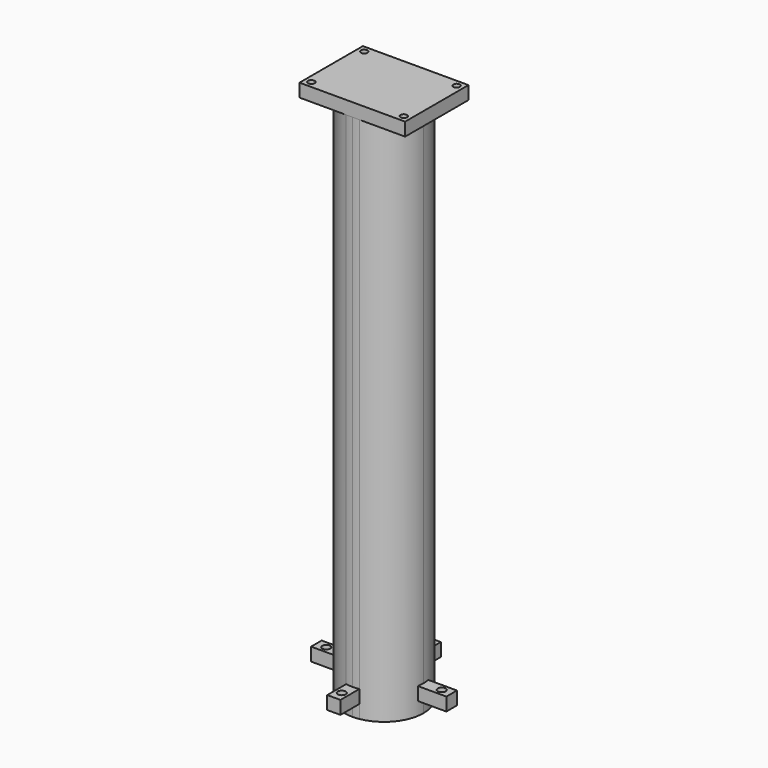
from build123d import *

# Parameters (mm, degrees)
F0_R     = 5
F1_DEPTH = 20
F2_DEPTH = 800
F5_DEPTH = 10
F6_DEPTH = 10
F0_R_2   = 6
F7_DEPTH = 956


# Not quite as in the source:
# - a feature names something its author has since deleted; it is built from what else it names


with BuildPart() as f1:
    # F0 (on Top) → F1 (new body)
    with BuildSketch(Plane.XY):
        with BuildLine():
            ThreePointArc((-59.160797831, 10), (-42.4264068712, 42.4264068712), (-10, 59.160797831))
            Line((-10, 59.160797831), (-10, 60))
            Line((-10, 60), (-80, 60))
            Line((-80, 60), (-80, 10))
            Line((-80, 10), (-59.160797831, 10))
        make_face()
        with Locations((-70, 50)):
            Circle(F0_R, mode=Mode.SUBTRACT)
        with BuildLine():
            ThreePointArc((59.160797831, -10), (59.7898313673, -5.0175756168), (60, 0))
            ThreePointArc((60, 0), (59.7898313673, 5.0175756168), (59.160797831, 10))
            ThreePointArc((59.160797831, 10), (42.4264068712, 42.4264068712), (10, 59.160797831))
            ThreePointArc((10, 59.160797831), (5.0175756193, 59.7898313671), (5e-09, 60))
            ThreePointArc((5e-09, 60), (-5.0175756143, 59.7898313675), (-10, 59.160797831))
            ThreePointArc((-10, 59.160797831), (-42.4264068712, 42.4264068712), (-59.160797831, 10))
            ThreePointArc((-59.160797831, 10), (-60, 0), (-59.160797831, -10))
            ThreePointArc((-59.160797831, -10), (-42.4264068712, -42.4264068712), (-10, -59.160797831))
            ThreePointArc((-10, -59.160797831), (-5.0175756489, -59.7898313646), (-6.44e-08, -60))
            ThreePointArc((-6.44e-08, -60), (5.0175755847, -59.78983137), (10, -59.160797831))
            ThreePointArc((10, -59.160797831), (42.4264068712, -42.4264068712), (59.160797831, -10))
        make_face()
        with BuildLine():
            ThreePointArc((10, 59.160797831), (42.4264068712, 42.4264068712), (59.160797831, 10))
            Line((59.160797831, 10), (80, 10))
            Line((80, 10), (80, 60))
            Line((80, 60), (10, 60))
            Line((10, 60), (10, 59.160797831))
        make_face()
        with Locations((70, 50)):
            Circle(F0_R, mode=Mode.SUBTRACT)
        with BuildLine():
            ThreePointArc((59.160797831, 10), (59.7898313673, 5.0175756168), (60, 0))
            ThreePointArc((60, 0), (59.7898313673, -5.0175756168), (59.160797831, -10))
            Line((59.160797831, -10), (80, -10))
            Line((80, -10), (80, 10))
            Line((80, 10), (59.160797831, 10))
        make_face()
        with BuildLine():
            Line((80, -10), (59.160797831, -10))
            ThreePointArc((59.160797831, -10), (42.4264068712, -42.4264068712), (10, -59.160797831))
            Line((10, -59.160797831), (10, -60))
            Line((10, -60), (80, -60))
            Line((80, -60), (80, -10))
        make_face()
        with Locations((70, -50)):
            Circle(F0_R, mode=Mode.SUBTRACT)
        with BuildLine():
            ThreePointArc((-59.160797831, -10), (-60, 0), (-59.160797831, 10))
            Line((-59.160797831, 10), (-80, 10))
            Line((-80, 10), (-80, -10))
            Line((-80, -10), (-59.160797831, -10))
        make_face()
        with BuildLine():
            Line((-10, -60), (-10, -59.160797831))
            ThreePointArc((-10, -59.160797831), (-42.4264068712, -42.4264068712), (-59.160797831, -10))
            Line((-59.160797831, -10), (-80, -10))
            Line((-80, -10), (-80, -60))
            Line((-80, -60), (-10, -60))
        make_face()
        with Locations((-70, -50)):
            Circle(F0_R, mode=Mode.SUBTRACT)
        with BuildLine():
            Line((-10, -60), (-6.44e-08, -60))
            ThreePointArc((-6.44e-08, -60), (-5.0175756489, -59.7898313646), (-10, -59.160797831))
            Line((-10, -59.160797831), (-10, -60))
        make_face()
        with BuildLine():
            Line((10, -60), (10, -59.160797831))
            ThreePointArc((10, -59.160797831), (5.0175755847, -59.78983137), (-6.44e-08, -60))
            Line((-6.44e-08, -60), (10, -60))
        make_face()
        with BuildLine():
            ThreePointArc((-10, 59.160797831), (-5.0175756143, 59.7898313675), (5e-09, 60))
            Line((5e-09, 60), (-10, 60))
            Line((-10, 60), (-10, 59.160797831))
        make_face()
        with BuildLine():
            ThreePointArc((5e-09, 60), (5.0175756193, 59.7898313671), (10, 59.160797831))
            Line((10, 59.160797831), (10, 60))
            Line((10, 60), (5e-09, 60))
        make_face()
    extrude(amount=F1_DEPTH)

    # F0 (on Top) → F2 (join)
    with BuildSketch(Plane.XY):
        with BuildLine():
            ThreePointArc((59.160797831, -10), (59.7898313673, -5.0175756168), (60, 0))
            ThreePointArc((60, 0), (59.7898313673, 5.0175756168), (59.160797831, 10))
            ThreePointArc((59.160797831, 10), (42.4264068712, 42.4264068712), (10, 59.160797831))
            ThreePointArc((10, 59.160797831), (5.0175756193, 59.7898313671), (5e-09, 60))
            ThreePointArc((5e-09, 60), (-5.0175756143, 59.7898313675), (-10, 59.160797831))
            ThreePointArc((-10, 59.160797831), (-42.4264068712, 42.4264068712), (-59.160797831, 10))
            ThreePointArc((-59.160797831, 10), (-60, 0), (-59.160797831, -10))
            ThreePointArc((-59.160797831, -10), (-42.4264068712, -42.4264068712), (-10, -59.160797831))
            ThreePointArc((-10, -59.160797831), (-5.0175756489, -59.7898313646), (-6.44e-08, -60))
            ThreePointArc((-6.44e-08, -60), (5.0175755847, -59.78983137), (10, -59.160797831))
            ThreePointArc((10, -59.160797831), (42.4264068712, -42.4264068712), (59.160797831, -10))
        make_face()
    extrude(amount=-F2_DEPTH)

    # F4 (on Right) → F5 (join, symmetric)
    with BuildSketch(Plane.YZ):
        Polygon((95, -760), (0, -760), (-95, -760), (-95, -780), (95, -780), align=None)
    extrude(amount=F5_DEPTH, both=True)

    # F3 (on Front) → F6 (join, symmetric)
    with BuildSketch(Plane.XZ):
        Polygon((102.5, -760), (0, -760), (-102.5, -760), (-102.5, -780), (102.5, -780), align=None)
    extrude(amount=F6_DEPTH, both=True)

    # F0 (on Top) → F7 (cut)
    with BuildSketch(Plane.XY):
        with Locations((0, 80)):
            Circle(F0_R_2)
        with Locations((0, -80)):
            Circle(F0_R_2)
        with Locations((87.5, 0)):
            Circle(F0_R_2)
        with Locations((-87.5, 0)):
            Circle(F0_R_2)
    extrude(amount=-F7_DEPTH, mode=Mode.SUBTRACT)


solid = f1.part
